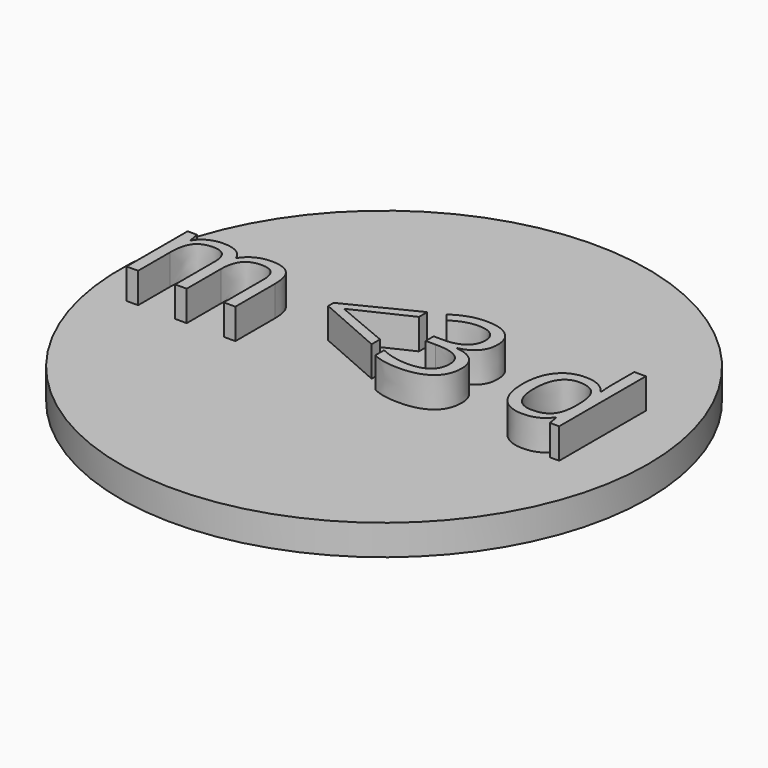
from build123d import *

# Parameters (mm, degrees)
F0_R         = 22.0853
F2_DEPTH     = 2.54
F3_TEXT_SIZE = 11.9297403014
F4_DEPTH     = 2.54


# Not quite as in the source:
# - a feature names something its author has since deleted; it is built from what else it names
# - Text() gives the source's letters only with a copy of the font that has no kerning and outlines rounded to 1/6400 em; it was checked with that copy


with BuildPart() as f2:
    # F0 (on Top) → F2 (new body)
    with BuildSketch(Plane.XY):
        Circle(F0_R)
    extrude(amount=F2_DEPTH)

    # F3 (on face) → F4 (join)
    with BuildSketch(Plane.XY.offset(2.54)):
        with Locations((-19.9755243957, -3.245477099)):
            Text('m <3 d', F3_TEXT_SIZE, font='Open Sans', text_align=(TextAlign.LEFT, TextAlign.BOTTOM))
    extrude(amount=F4_DEPTH)


solid = f2.part
